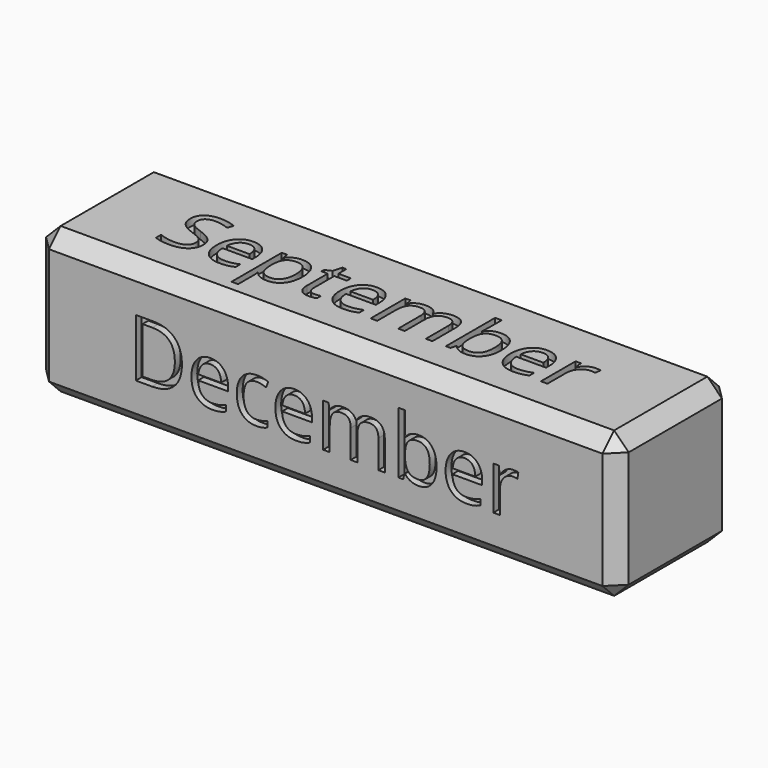
from build123d import *

# Parameters (mm, degrees)
F0_W          = 101.6
F0_H          = 25.4
F1_DEPTH      = 12.7
F1_DEPTH_BACK = 12.7
F2_SIZE       = 2.54
F3_TEXT_SIZE  = 14.1111111111
F4_DEPTH      = 1.27
F5_TEXT_SIZE  = 14.1111111111
F6_DEPTH      = 1.27
F7_TEXT_SIZE  = 14.1111111111
F8_DEPTH      = 1.27
F9_TEXT_SIZE  = 14.1111111111
F10_DEPTH     = 1.27


# Not quite as in the source:
# - Text() gives the source's letters only with a copy of the font that has no kerning and outlines rounded to 1/6400 em; it was checked with that copy


with BuildPart() as f1:
    # F0 (on Top) → F1 (new body, two sides)
    with BuildSketch(Plane.XY) as f1_sk:
        Rectangle(F0_W, F0_H)
    extrude(amount=F1_DEPTH)
    extrude(f1_sk.sketch, amount=-F1_DEPTH_BACK)

    # F2
    f2_edges = [f1.edges().sort_by_distance(p)[0] for p in [
        (-50.8, 0, 12.7),
        (-50.8, -12.7, 0),
        (-50.8, 0, -12.7),
        (-50.8, 12.7, 0),
        (50.8, 0, 12.7),
        (0, 12.7, 12.7),
        (0, -12.7, 12.7),
        (50.8, -12.7, 0),
        (0, -12.7, -12.7),
        (50.8, 12.7, 0),
        (50.8, 0, -12.7),
        (0, 12.7, -12.7),
    ]]
    chamfer(f2_edges, length=F2_SIZE)

    # F3 (on face) → F4 (cut)
    with BuildSketch(Plane.XY.offset(12.7)):
        with Locations((-36.6877864583, -5.08)):
            Text('September', F3_TEXT_SIZE, font='Open Sans', text_align=(TextAlign.LEFT, TextAlign.BOTTOM))
    extrude(amount=-F4_DEPTH, mode=Mode.SUBTRACT)

    # F5 (on face) → F6 (cut)
    with BuildSketch(Plane(origin=(0, 12.7, 0), x_dir=(-1, 0, 0), z_dir=(0, 1, 0))):
        with Locations(Location((27.12640625, 5.08), (0, 0, -180))):
            Text('October', F5_TEXT_SIZE, font='Open Sans', text_align=(TextAlign.LEFT, TextAlign.BOTTOM))
    extrude(amount=-F6_DEPTH, mode=Mode.SUBTRACT)

    # F7 (on face) → F8 (cut)
    with BuildSketch(Plane(origin=(0, 0, -12.7), x_dir=(1, 0, 0), z_dir=(0, 0, -1))):
        with Locations((-35.1576128472, -5.08)):
            Text('November', F7_TEXT_SIZE, font='Open Sans', text_align=(TextAlign.LEFT, TextAlign.BOTTOM))
    extrude(amount=-F8_DEPTH, mode=Mode.SUBTRACT)

    # F9 (on face) → F10 (cut)
    with BuildSketch(Plane.XZ.offset(12.7)):
        with Locations((-34.5038715278, -5.08)):
            Text('December', F9_TEXT_SIZE, font='Open Sans', text_align=(TextAlign.LEFT, TextAlign.BOTTOM))
    extrude(amount=-F10_DEPTH, mode=Mode.SUBTRACT)


solid = f1.part
